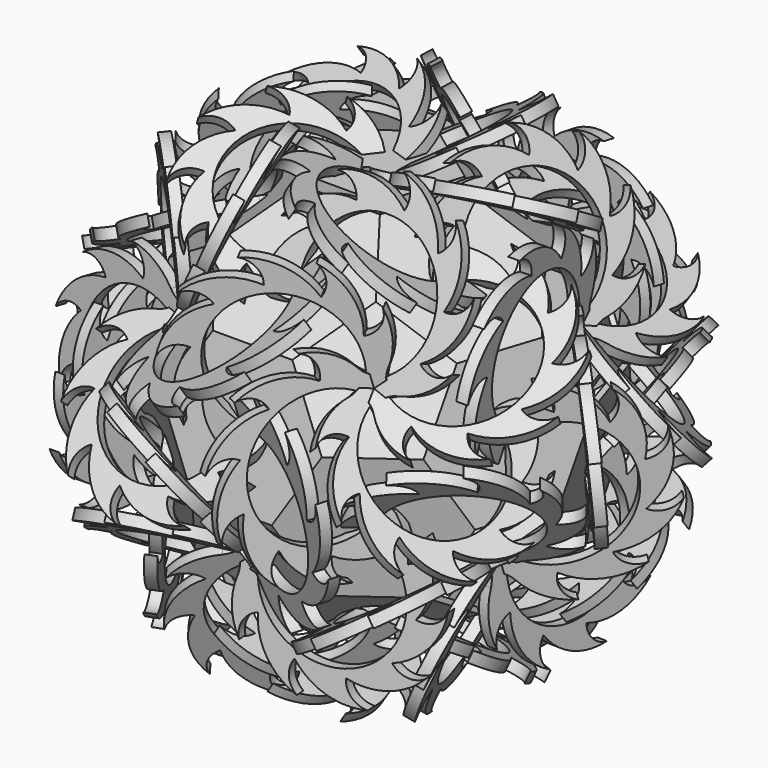
from build123d import *

# Parameters (mm, degrees)
F2_DEPTH  = 1
F3_DEPTH  = 1
F4_ANGLE  = -37.377368
F6_COUNT  = 5
F6_ANGLE  = 288
F9_DEPTH  = 2
F10_R     = 5
F12_ANGLE = 65
F13_COUNT = 5
F13_ANGLE = 288
F15_COUNT = 3
F15_ANGLE = 240
F16_COUNT = 5
F16_ANGLE = 288
F17_COUNT = 2
F17_ANGLE = 120
F18_COUNT = 3
F18_ANGLE = 240
F22_COUNT = 3
F22_ANGLE = 144
F26_COUNT = 3
F26_ANGLE = 144
F29_COUNT = 2
F29_ANGLE = 120
F32_COUNT = 3
F32_ANGLE = 144
F36_COUNT = 3
F36_ANGLE = 240
F40_COUNT = 3
F40_ANGLE = 144
F44_COUNT = 3
F44_ANGLE = 144
F48_COUNT = 2
F48_ANGLE = 120
F52_COUNT = 2
F52_ANGLE = 120
F56_COUNT = 2
F56_ANGLE = 120
F60_COUNT = 2
F60_ANGLE = 120
F65_DEPTH = 2


with BuildPart() as f2:
    # F0 (on Top) → F2 (new body)
    with BuildSketch(Plane.XY):
        Polygon((0, -10.3228644035), (7.5, -10.3228644035), (12.1352549156, 3.9429833409), (0, 12.7597621253), align=None)
        Polygon((-7.5, -10.3228644035), (0, -10.3228644035), (0, 12.7597621253), (-12.1352549156, 3.9429833409), align=None)
    extrude(amount=-F2_DEPTH)


with BuildPart() as f3:
    # F1 (on Top) → F3 (new body)
    with BuildSketch(Plane.XY):
        Polygon((32.2091731064, -18.3513614234), (36.844428022, -4.085513679), (26.8074689266, 7.0616587032), (12.1352549156, 3.9429833409), (7.5, -10.3228644035), (17.5369590954, -21.4700367857), align=None)
    extrude(amount=-F3_DEPTH)


with BuildPart() as f3_1:
    # F4: moved
    add(f3.part.rotate(Axis((9.8176274578, -3.1899405313, 0), (-0.3090169944, -0.9510565163, 0)), F4_ANGLE))


with BuildPart() as f6_1:
    # F6: instance of F3
    add(f3_1.part.rotate(Axis((0, 0, 3.8664315362), (0, 0, 1)), 1 * F6_ANGLE / (F6_COUNT - 1)))


with BuildPart() as f6_2:
    # F6: instance of F3
    add(f3_1.part.rotate(Axis((0, 0, 3.8664315362), (0, 0, 1)), 2 * F6_ANGLE / (F6_COUNT - 1)))


with BuildPart() as f6_3:
    # F6: instance of F3
    add(f3_1.part.rotate(Axis((0, 0, 3.8664315362), (0, 0, 1)), 3 * F6_ANGLE / (F6_COUNT - 1)))


with BuildPart() as f6_4:
    # F6: instance of F3
    add(f3_1.part.rotate(Axis((0, 0, 3.8664315362), (0, 0, 1)), 4 * F6_ANGLE / (F6_COUNT - 1)))


with BuildPart() as f9:
    # F8 (on Right) → F9 (new body)
    with BuildSketch(Plane.YZ):
        with BuildLine():
            ThreePointArc((-20.0381562793, -7.4218225341), (-18.0432138806, 14.7456768661), (-1.371596125, 0))
            ThreePointArc((-1.371596125, 0), (1.2710572909, -2.1110060804), (1.0658705895, 1.265065922))
            ThreePointArc((1.0658705895, 1.265065922), (3.462744203, 7.3677169674), (2.5001799222, 13.8531485572))
            ThreePointArc((2.5001799222, 13.8531485572), (1.8396441745, 10.7438611605), (-0.8004298525, 8.9735547684))
            ThreePointArc((-0.8004298525, 8.9735547684), (-2.1304901639, 15.9377846017), (-6.983453041, 21.1067602176))
            ThreePointArc((-6.983453041, 21.1067602176), (-5.7243130519, 18.2607184854), (-6.7542303289, 15.3239417734))
            ThreePointArc((-6.7542303289, 15.3239417734), (-11.923743314, 20.1763322255), (-18.8881203911, 21.5056213332))
            ThreePointArc((-18.8881203911, 21.5056213332), (-16.196593384, 19.9432291213), (-15.3036199233, 16.9619566661))
            ThreePointArc((-15.3036199233, 16.9619566661), (-22.3380073271, 17.8490595111), (-28.7536432712, 14.8309188523))
            ThreePointArc((-28.7536432712, 14.8309188523), (-25.6578010812, 15.1489568819), (-23.1830223937, 13.2619334316))
            ThreePointArc((-23.1830223937, 13.2619334316), (-29.3953873179, 9.8449055341), (-32.8117272579, 3.6321622578))
            ThreePointArc((-32.8117272579, 3.6321622578), (-30.4940763777, 5.7091508113), (-27.3827738075, 5.6371551864))
            ThreePointArc((-27.3827738075, 5.6371551864), (-30.4002040016, -0.7788149372), (-29.5123221974, -7.813104063))
            ThreePointArc((-29.5123221974, -7.813104063), (-28.8581264893, -4.7705040188), (-26.2987118688, -2.9999719366))
            ThreePointArc((-26.2987118688, -2.9999719366), (-26.0274642787, -7.0575500385), (-24.4889350399, -10.821914937))
            ThreePointArc((-24.4889350399, -10.821914937), (-20.5634994581, -11.3472581158), (-20.0381562793, -7.4218225341))
        make_face()
    extrude(amount=-F9_DEPTH)

    # F10
    f10_edges = [f9.edges().sort_by_distance(p)[0] for p in [
        (-1, 1.065871, 1.265066),
    ]]
    fillet(f10_edges, radius=F10_R)


with BuildPart() as f9_1:
    # F12: moved
    add(f9.part.rotate(Axis((0, -10.3228644132, -3.9429833282), (0, -0.9341723595, -0.3568220885)), F12_ANGLE))


with BuildPart() as f13_1:
    # F13: instance of F9
    add(f9_1.part.rotate(Axis((0, 0, 14.2103461549), (0, 0, 1)), 1 * F13_ANGLE / (F13_COUNT - 1)))


with BuildPart() as f13_2:
    # F13: instance of F9
    add(f9_1.part.rotate(Axis((0, 0, 14.2103461549), (0, 0, 1)), 2 * F13_ANGLE / (F13_COUNT - 1)))


with BuildPart() as f13_3:
    # F13: instance of F9
    add(f9_1.part.rotate(Axis((0, 0, 14.2103461549), (0, 0, 1)), 3 * F13_ANGLE / (F13_COUNT - 1)))


with BuildPart() as f13_4:
    # F13: instance of F9
    add(f9_1.part.rotate(Axis((0, 0, 14.2103461549), (0, 0, 1)), 4 * F13_ANGLE / (F13_COUNT - 1)))


with BuildPart() as f15_1:
    # F15: instance of F9
    add(f9_1.part.rotate(Axis((0, -25.3455492518, -1.7338218178), (0, -0.6070619963, 0.7946544738)), 1 * F15_ANGLE / (F15_COUNT - 1)))


with BuildPart() as f15_2:
    # F15: instance of F9
    add(f9_1.part.rotate(Axis((0, -25.3455492518, -1.7338218178), (0, -0.6070619963, 0.7946544738)), 2 * F15_ANGLE / (F15_COUNT - 1)))


with BuildPart() as f16_1:
    # F16: instance of F15_2
    add(f15_2.part.rotate(Axis((0, 0, 14.2103461549), (0, 0, 1)), 1 * F16_ANGLE / (F16_COUNT - 1)))


with BuildPart() as f16_2:
    # F16: instance of F15_2
    add(f15_2.part.rotate(Axis((0, 0, 14.2103461549), (0, 0, 1)), 2 * F16_ANGLE / (F16_COUNT - 1)))


with BuildPart() as f16_3:
    # F16: instance of F15_2
    add(f15_2.part.rotate(Axis((0, 0, 14.2103461549), (0, 0, 1)), 3 * F16_ANGLE / (F16_COUNT - 1)))


with BuildPart() as f16_4:
    # F16: instance of F15_2
    add(f15_2.part.rotate(Axis((0, 0, 14.2103461549), (0, 0, 1)), 4 * F16_ANGLE / (F16_COUNT - 1)))


with BuildPart() as f16_5:
    # F16: instance of F15_1
    add(f15_1.part.rotate(Axis((0, 0, 14.2103461549), (0, 0, 1)), 1 * F16_ANGLE / (F16_COUNT - 1)))


with BuildPart() as f16_6:
    # F16: instance of F15_1
    add(f15_1.part.rotate(Axis((0, 0, 14.2103461549), (0, 0, 1)), 2 * F16_ANGLE / (F16_COUNT - 1)))


with BuildPart() as f16_7:
    # F16: instance of F15_1
    add(f15_1.part.rotate(Axis((0, 0, 14.2103461549), (0, 0, 1)), 3 * F16_ANGLE / (F16_COUNT - 1)))


with BuildPart() as f16_8:
    # F16: instance of F15_1
    add(f15_1.part.rotate(Axis((0, 0, 14.2103461549), (0, 0, 1)), 4 * F16_ANGLE / (F16_COUNT - 1)))


with BuildPart() as f17_1:
    # F17: instance of F3
    add(f3_1.part.rotate(Axis((0, -25.3455492518, -1.7338218178), (0, 0.6070619963, -0.7946544738)), 1 * F17_ANGLE / (F17_COUNT - 1)))


with BuildPart() as f17_2:
    # F17: instance of F16_5
    add(f16_5.part.rotate(Axis((0, -25.3455492518, -1.7338218178), (0, 0.6070619963, -0.7946544738)), 1 * F17_ANGLE / (F17_COUNT - 1)))


with BuildPart() as f17_3:
    # F17: instance of F13_1
    add(f13_1.part.rotate(Axis((0, -25.3455492518, -1.7338218178), (0, 0.6070619963, -0.7946544738)), 1 * F17_ANGLE / (F17_COUNT - 1)))


with BuildPart() as f17_4:
    # F17: instance of F16_1
    add(f16_1.part.rotate(Axis((0, -25.3455492518, -1.7338218178), (0, 0.6070619963, -0.7946544738)), 1 * F17_ANGLE / (F17_COUNT - 1)))


with BuildPart() as f18_1:
    # F18: instance of F2
    add(f2.part.rotate(Axis((0, -25.3455492518, -1.7338218178), (0, -0.6070619963, 0.7946544738)), 1 * F18_ANGLE / (F18_COUNT - 1)))


with BuildPart() as f18_2:
    # F18: instance of F2
    add(f2.part.rotate(Axis((0, -25.3455492518, -1.7338218178), (0, -0.6070619963, 0.7946544738)), 2 * F18_ANGLE / (F18_COUNT - 1)))


with BuildPart() as f18_3:
    # F18: instance of F13_2
    add(f13_2.part.rotate(Axis((0, -25.3455492518, -1.7338218178), (0, -0.6070619963, 0.7946544738)), 1 * F18_ANGLE / (F18_COUNT - 1)))


with BuildPart() as f18_4:
    # F18: instance of F13_2
    add(f13_2.part.rotate(Axis((0, -25.3455492518, -1.7338218178), (0, -0.6070619963, 0.7946544738)), 2 * F18_ANGLE / (F18_COUNT - 1)))


with BuildPart() as f18_5:
    # F18: instance of F13_3
    add(f13_3.part.rotate(Axis((0, -25.3455492518, -1.7338218178), (0, -0.6070619963, 0.7946544738)), 1 * F18_ANGLE / (F18_COUNT - 1)))


with BuildPart() as f18_6:
    # F18: instance of F13_3
    add(f13_3.part.rotate(Axis((0, -25.3455492518, -1.7338218178), (0, -0.6070619963, 0.7946544738)), 2 * F18_ANGLE / (F18_COUNT - 1)))


with BuildPart() as f22_1:
    # F22: instance of F17_1
    add(f17_1.part.rotate(Axis((-18.9711930891, -26.1116072266, -18.7737157723), (0.5257311104, 0.7236067968, -0.4472135991)), 1 * F22_ANGLE / (F22_COUNT - 1)))


with BuildPart() as f22_2:
    # F22: instance of F17_1
    add(f17_1.part.rotate(Axis((-18.9711930891, -26.1116072266, -18.7737157723), (0.5257311104, 0.7236067968, -0.4472135991)), 2 * F22_ANGLE / (F22_COUNT - 1)))


with BuildPart() as f22_3:
    # F22: instance of F17_3
    add(f17_3.part.rotate(Axis((-18.9711930891, -26.1116072266, -18.7737157723), (0.5257311104, 0.7236067968, -0.4472135991)), 1 * F22_ANGLE / (F22_COUNT - 1)))


with BuildPart() as f22_4:
    # F22: instance of F17_3
    add(f17_3.part.rotate(Axis((-18.9711930891, -26.1116072266, -18.7737157723), (0.5257311104, 0.7236067968, -0.4472135991)), 2 * F22_ANGLE / (F22_COUNT - 1)))


with BuildPart() as f22_5:
    # F22: instance of F17_4
    add(f17_4.part.rotate(Axis((-18.9711930891, -26.1116072266, -18.7737157723), (0.5257311104, 0.7236067968, -0.4472135991)), 1 * F22_ANGLE / (F22_COUNT - 1)))


with BuildPart() as f22_6:
    # F22: instance of F17_4
    add(f17_4.part.rotate(Axis((-18.9711930891, -26.1116072266, -18.7737157723), (0.5257311104, 0.7236067968, -0.4472135991)), 2 * F22_ANGLE / (F22_COUNT - 1)))


with BuildPart() as f22_7:
    # F22: instance of F17_2
    add(f17_2.part.rotate(Axis((-18.9711930891, -26.1116072266, -18.7737157723), (0.5257311104, 0.7236067968, -0.4472135991)), 1 * F22_ANGLE / (F22_COUNT - 1)))


with BuildPart() as f22_8:
    # F22: instance of F17_2
    add(f17_2.part.rotate(Axis((-18.9711930891, -26.1116072266, -18.7737157723), (0.5257311104, 0.7236067968, -0.4472135991)), 2 * F22_ANGLE / (F22_COUNT - 1)))


with BuildPart() as f26_1:
    # F26: instance of F3
    add(f3_1.part.rotate(Axis((20.2758098134, -27.9072581024, -17.6639424888), (-0.5257311104, 0.7236067968, -0.4472135991)), 1 * F26_ANGLE / (F26_COUNT - 1)))


with BuildPart() as f26_2:
    # F26: instance of F3
    add(f3_1.part.rotate(Axis((20.2758098134, -27.9072581024, -17.6639424888), (-0.5257311104, 0.7236067968, -0.4472135991)), 2 * F26_ANGLE / (F26_COUNT - 1)))


with BuildPart() as f26_3:
    # F26: instance of F16_1
    add(f16_1.part.rotate(Axis((20.2758098134, -27.9072581024, -17.6639424888), (-0.5257311104, 0.7236067968, -0.4472135991)), 1 * F26_ANGLE / (F26_COUNT - 1)))


with BuildPart() as f26_4:
    # F26: instance of F16_1
    add(f16_1.part.rotate(Axis((20.2758098134, -27.9072581024, -17.6639424888), (-0.5257311104, 0.7236067968, -0.4472135991)), 2 * F26_ANGLE / (F26_COUNT - 1)))


with BuildPart() as f26_5:
    # F26: instance of F13_1
    add(f13_1.part.rotate(Axis((20.2758098134, -27.9072581024, -17.6639424888), (-0.5257311104, 0.7236067968, -0.4472135991)), 1 * F26_ANGLE / (F26_COUNT - 1)))


with BuildPart() as f26_6:
    # F26: instance of F13_1
    add(f13_1.part.rotate(Axis((20.2758098134, -27.9072581024, -17.6639424888), (-0.5257311104, 0.7236067968, -0.4472135991)), 2 * F26_ANGLE / (F26_COUNT - 1)))


with BuildPart() as f26_7:
    # F26: instance of F16_5
    add(f16_5.part.rotate(Axis((20.2758098134, -27.9072581024, -17.6639424888), (-0.5257311104, 0.7236067968, -0.4472135991)), 1 * F26_ANGLE / (F26_COUNT - 1)))


with BuildPart() as f26_8:
    # F26: instance of F16_5
    add(f16_5.part.rotate(Axis((20.2758098134, -27.9072581024, -17.6639424888), (-0.5257311104, 0.7236067968, -0.4472135991)), 2 * F26_ANGLE / (F26_COUNT - 1)))


with BuildPart() as f29_1:
    # F29: instance of F18_2
    add(f18_2.part.rotate(Axis((0, -40.5030693029, -27.1761785704), (0, 0.9822469455, -0.1875924789)), 1 * F29_ANGLE / (F29_COUNT - 1)))


with BuildPart() as f32_1:
    # F32: instance of F26_2
    add(f26_2.part.rotate(Axis((0, -41.1465715097, -55.4848620892), (0, 0.8944271941, 0.4472135893)), 1 * F32_ANGLE / (F32_COUNT - 1)))


with BuildPart() as f32_2:
    # F32: instance of F26_2
    add(f26_2.part.rotate(Axis((0, -41.1465715097, -55.4848620892), (0, 0.8944271941, 0.4472135893)), 2 * F32_ANGLE / (F32_COUNT - 1)))


with BuildPart() as f32_3:
    # F32: instance of F26_4
    add(f26_4.part.rotate(Axis((0, -41.1465715097, -55.4848620892), (0, 0.8944271941, 0.4472135893)), 1 * F32_ANGLE / (F32_COUNT - 1)))


with BuildPart() as f32_4:
    # F32: instance of F26_4
    add(f26_4.part.rotate(Axis((0, -41.1465715097, -55.4848620892), (0, 0.8944271941, 0.4472135893)), 2 * F32_ANGLE / (F32_COUNT - 1)))


with BuildPart() as f32_5:
    # F32: instance of F26_6
    add(f26_6.part.rotate(Axis((0, -41.1465715097, -55.4848620892), (0, 0.8944271941, 0.4472135893)), 1 * F32_ANGLE / (F32_COUNT - 1)))


with BuildPart() as f32_6:
    # F32: instance of F26_6
    add(f26_6.part.rotate(Axis((0, -41.1465715097, -55.4848620892), (0, 0.8944271941, 0.4472135893)), 2 * F32_ANGLE / (F32_COUNT - 1)))


with BuildPart() as f32_7:
    # F32: instance of F18_4
    add(f18_4.part.rotate(Axis((0, -41.1465715097, -55.4848620892), (0, 0.8944271941, 0.4472135893)), 1 * F32_ANGLE / (F32_COUNT - 1)))


with BuildPart() as f32_8:
    # F32: instance of F18_4
    add(f18_4.part.rotate(Axis((0, -41.1465715097, -55.4848620892), (0, 0.8944271941, 0.4472135893)), 2 * F32_ANGLE / (F32_COUNT - 1)))


with BuildPart() as f36_1:
    # F36: instance of F2
    add(f2.part.rotate(Axis((-17.4030966331, 23.953307566, 3.8456892929), (0.3568220886, -0.4911234716, -0.7946544738)), 1 * F36_ANGLE / (F36_COUNT - 1)))


with BuildPart() as f36_2:
    # F36: instance of F2
    add(f2.part.rotate(Axis((-17.4030966331, 23.953307566, 3.8456892929), (0.3568220886, -0.4911234716, -0.7946544738)), 2 * F36_ANGLE / (F36_COUNT - 1)))


with BuildPart() as f40_1:
    # F40: instance of F22_2
    add(f22_2.part.rotate(Axis((-43.9943598437, 14.2946340797, -11.7823727251), (0.8506508064, -0.2763932025, -0.4472135991)), 1 * F40_ANGLE / (F40_COUNT - 1)))


with BuildPart() as f40_2:
    # F40: instance of F22_2
    add(f22_2.part.rotate(Axis((-43.9943598437, 14.2946340797, -11.7823727251), (0.8506508064, -0.2763932025, -0.4472135991)), 2 * F40_ANGLE / (F40_COUNT - 1)))


with BuildPart() as f40_3:
    # F40: instance of F22_6
    add(f22_6.part.rotate(Axis((-43.9943598437, 14.2946340797, -11.7823727251), (0.8506508064, -0.2763932025, -0.4472135991)), 1 * F40_ANGLE / (F40_COUNT - 1)))


with BuildPart() as f40_4:
    # F40: instance of F22_6
    add(f22_6.part.rotate(Axis((-43.9943598437, 14.2946340797, -11.7823727251), (0.8506508064, -0.2763932025, -0.4472135991)), 2 * F40_ANGLE / (F40_COUNT - 1)))


with BuildPart() as f40_5:
    # F40: instance of F22_4
    add(f22_4.part.rotate(Axis((-43.9943598437, 14.2946340797, -11.7823727251), (0.8506508064, -0.2763932025, -0.4472135991)), 1 * F40_ANGLE / (F40_COUNT - 1)))


with BuildPart() as f40_6:
    # F40: instance of F22_4
    add(f22_4.part.rotate(Axis((-43.9943598437, 14.2946340797, -11.7823727251), (0.8506508064, -0.2763932025, -0.4472135991)), 2 * F40_ANGLE / (F40_COUNT - 1)))


with BuildPart() as f40_7:
    # F40: instance of F18_3
    add(f18_3.part.rotate(Axis((-43.9943598437, 14.2946340797, -11.7823727251), (0.8506508064, -0.2763932025, -0.4472135991)), 1 * F40_ANGLE / (F40_COUNT - 1)))


with BuildPart() as f40_8:
    # F40: instance of F18_3
    add(f18_3.part.rotate(Axis((-43.9943598437, 14.2946340797, -11.7823727251), (0.8506508064, -0.2763932025, -0.4472135991)), 2 * F40_ANGLE / (F40_COUNT - 1)))


with BuildPart() as f44_1:
    # F44: instance of F40_2
    add(f40_2.part.rotate(Axis((1.534e-07, 54.8190866503, -7.5020330917), (-6.9e-09, -0.8944271892, -0.4472135991)), 1 * F44_ANGLE / (F44_COUNT - 1)))


with BuildPart() as f44_2:
    # F44: instance of F40_2
    add(f40_2.part.rotate(Axis((1.534e-07, 54.8190866503, -7.5020330917), (-6.9e-09, -0.8944271892, -0.4472135991)), 2 * F44_ANGLE / (F44_COUNT - 1)))


with BuildPart() as f44_3:
    # F44: instance of F40_6
    add(f40_6.part.rotate(Axis((1.534e-07, 54.8190866503, -7.5020330917), (-6.9e-09, -0.8944271892, -0.4472135991)), 1 * F44_ANGLE / (F44_COUNT - 1)))


with BuildPart() as f44_4:
    # F44: instance of F40_6
    add(f40_6.part.rotate(Axis((1.534e-07, 54.8190866503, -7.5020330917), (-6.9e-09, -0.8944271892, -0.4472135991)), 2 * F44_ANGLE / (F44_COUNT - 1)))


with BuildPart() as f44_5:
    # F44: instance of F40_8
    add(f40_8.part.rotate(Axis((1.534e-07, 54.8190866503, -7.5020330917), (-6.9e-09, -0.8944271892, -0.4472135991)), 1 * F44_ANGLE / (F44_COUNT - 1)))


with BuildPart() as f44_6:
    # F44: instance of F40_8
    add(f40_8.part.rotate(Axis((1.534e-07, 54.8190866503, -7.5020330917), (-6.9e-09, -0.8944271892, -0.4472135991)), 2 * F44_ANGLE / (F44_COUNT - 1)))


with BuildPart() as f44_7:
    # F44: instance of F40_4
    add(f40_4.part.rotate(Axis((1.534e-07, 54.8190866503, -7.5020330917), (-6.9e-09, -0.8944271892, -0.4472135991)), 1 * F44_ANGLE / (F44_COUNT - 1)))


with BuildPart() as f44_8:
    # F44: instance of F40_4
    add(f40_4.part.rotate(Axis((1.534e-07, 54.8190866503, -7.5020330917), (-6.9e-09, -0.8944271892, -0.4472135991)), 2 * F44_ANGLE / (F44_COUNT - 1)))


with BuildPart() as f48_1:
    # F48: instance of F22_2
    add(f22_2.part.rotate(Axis((-45.320051719, 14.7253777202, -44.0123603845), (0.9341723533, -0.3035310175, 0.1875924726)), 1 * F48_ANGLE / (F48_COUNT - 1)))


with BuildPart() as f48_2:
    # F48: instance of F22_4
    add(f22_4.part.rotate(Axis((-45.320051719, 14.7253777202, -44.0123603845), (0.9341723533, -0.3035310175, 0.1875924726)), 1 * F48_ANGLE / (F48_COUNT - 1)))


with BuildPart() as f48_3:
    # F48: instance of F22_6
    add(f22_6.part.rotate(Axis((-45.320051719, 14.7253777202, -44.0123603845), (0.9341723533, -0.3035310175, 0.1875924726)), 1 * F48_ANGLE / (F48_COUNT - 1)))


with BuildPart() as f48_4:
    # F48: instance of F18_3
    add(f18_3.part.rotate(Axis((-45.320051719, 14.7253777202, -44.0123603845), (0.9341723533, -0.3035310175, 0.1875924726)), 1 * F48_ANGLE / (F48_COUNT - 1)))


with BuildPart() as f52_1:
    # F52: instance of F16_5
    add(f16_5.part.rotate(Axis((51.1630279448, -16.6238756598, -24.6374564773), (-0.9341723577, 0.3035310035, -0.1875924733)), 1 * F52_ANGLE / (F52_COUNT - 1)))


with BuildPart() as f52_2:
    # F52: instance of F13_1
    add(f13_1.part.rotate(Axis((51.1630279448, -16.6238756598, -24.6374564773), (-0.9341723577, 0.3035310035, -0.1875924733)), 1 * F52_ANGLE / (F52_COUNT - 1)))


with BuildPart() as f52_3:
    # F52: instance of F16_1
    add(f16_1.part.rotate(Axis((51.1630279448, -16.6238756598, -24.6374564773), (-0.9341723577, 0.3035310035, -0.1875924733)), 1 * F52_ANGLE / (F52_COUNT - 1)))


with BuildPart() as f52_4:
    # F52: instance of F3
    add(f3_1.part.rotate(Axis((51.1630279448, -16.6238756598, -24.6374564773), (-0.9341723577, 0.3035310035, -0.1875924733)), 1 * F52_ANGLE / (F52_COUNT - 1)))


with BuildPart() as f56_1:
    # F56: instance of F26_2
    add(f26_2.part.rotate(Axis((20.2389789509, -27.8565650407, -79.9844450272), (-0.3568220897, 0.4911234788, 0.7946544689)), 1 * F56_ANGLE / (F56_COUNT - 1)))


with BuildPart() as f56_2:
    # F56: instance of F26_4
    add(f26_4.part.rotate(Axis((20.2389789509, -27.8565650407, -79.9844450272), (-0.3568220897, 0.4911234788, 0.7946544689)), 1 * F56_ANGLE / (F56_COUNT - 1)))


with BuildPart() as f56_3:
    # F56: instance of F26_6
    add(f26_6.part.rotate(Axis((20.2389789509, -27.8565650407, -79.9844450272), (-0.3568220897, 0.4911234788, 0.7946544689)), 1 * F56_ANGLE / (F56_COUNT - 1)))


with BuildPart() as f56_4:
    # F56: instance of F18_4
    add(f18_4.part.rotate(Axis((20.2389789509, -27.8565650407, -79.9844450272), (-0.3568220897, 0.4911234788, 0.7946544689)), 1 * F56_ANGLE / (F56_COUNT - 1)))


with BuildPart() as f60_1:
    # F60: instance of F52_4
    add(f52_4.part.rotate(Axis((24.2012826257, 7.8634731584, -68.221784607), (-0.5773502692, -0.1875924683, 0.7946544737)), 1 * F60_ANGLE / (F60_COUNT - 1)))


with BuildPart() as f60_2:
    # F60: instance of F52_3
    add(f52_3.part.rotate(Axis((24.2012826257, 7.8634731584, -68.221784607), (-0.5773502692, -0.1875924683, 0.7946544737)), 1 * F60_ANGLE / (F60_COUNT - 1)))


with BuildPart() as f60_3:
    # F60: instance of F52_1
    add(f52_1.part.rotate(Axis((24.2012826257, 7.8634731584, -68.221784607), (-0.5773502692, -0.1875924683, 0.7946544737)), 1 * F60_ANGLE / (F60_COUNT - 1)))


with BuildPart() as f60_4:
    # F60: instance of F52_2
    add(f52_2.part.rotate(Axis((24.2012826257, 7.8634731584, -68.221784607), (-0.5773502692, -0.1875924683, 0.7946544737)), 1 * F60_ANGLE / (F60_COUNT - 1)))


with BuildPart() as f2_1:
    add(f2.part)

    # F65 (add): a face of the model
    f65_faces = [f2_1.faces().sort_by_distance(p)[0] for p in [
        (0, 0, 0),
    ]]
    extrude(f65_faces, amount=F65_DEPTH)


solid = Compound([f3_1.part, f6_1.part, f6_2.part, f6_3.part, f6_4.part, f9_1.part, f13_1.part, f13_2.part, f13_3.part, f13_4.part, f15_1.part, f15_2.part, f16_1.part, f16_2.part, f16_3.part, f16_4.part, f16_5.part, f16_6.part, f16_7.part, f16_8.part, f17_1.part, f17_2.part, f17_3.part, f17_4.part, f18_1.part, f18_2.part, f18_3.part, f18_4.part, f18_5.part, f18_6.part, f22_1.part, f22_2.part, f22_3.part, f22_4.part, f22_5.part, f22_6.part, f26_1.part, f26_2.part, f26_3.part, f26_4.part, f26_5.part, f26_6.part, f29_1.part, f32_1.part, f32_2.part, f32_3.part, f32_4.part, f32_5.part, f32_6.part, f32_7.part, f32_8.part, f36_1.part, f36_2.part, f40_1.part, f40_2.part, f40_3.part, f40_4.part, f40_5.part, f40_6.part, f40_7.part, f40_8.part, f44_1.part, f44_2.part, f44_3.part, f44_4.part, f44_5.part, f44_6.part, f44_7.part, f44_8.part, f48_1.part, f48_2.part, f48_3.part, f48_4.part, f52_1.part, f52_2.part, f52_3.part, f52_4.part, f56_1.part, f56_2.part, f56_3.part, f56_4.part, f60_1.part, f60_2.part, f60_3.part, f60_4.part, f2_1.part])
